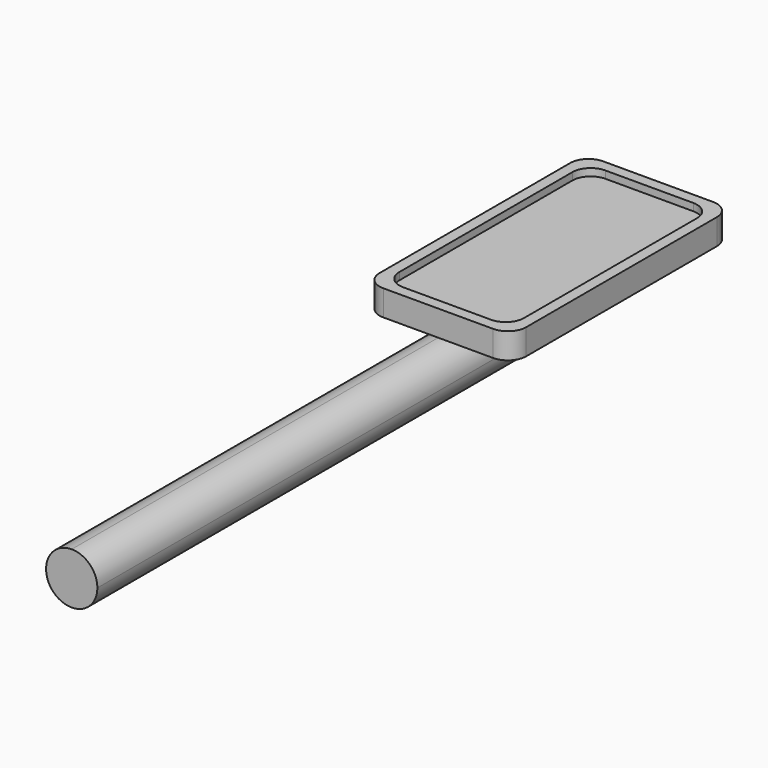
from build123d import *

# Parameters (mm, degrees)
F0_W     = 7
F0_H     = 200
F1_DEPTH = 7
F3_R     = 6.99999
F5_W     = 34
F5_H     = 69
F6_DEPTH = 5
F5_W_2   = 40
F5_H_2   = 75
F7_DEPTH = 7
F8_R     = 5
F9_R     = 5
F10_R    = 5
F11_R    = 5


# Not quite as in the source:
# - a fillet or chamfer is up to 0.001 mm smaller than in the source, because OpenCascade refuses the exact size


with BuildPart() as f1:
    # F0 (on Top) → F1 (new body)
    with BuildSketch(Plane.XY):
        with Locations((3.5, 0)):
            Rectangle(F0_W, F0_H)
    extrude(amount=F1_DEPTH)

    # F0 (on Top) → F2 (revolve)
    with BuildSketch(Plane.XY):
        with Locations((3.5, 0)):
            Rectangle(F0_W, F0_H)
    revolve(axis=Axis((0, 0, 0), (0, -1, 0)))

    # F3 (radius 7 in the source; OpenCascade refuses exactly that, so slightly less here)
    f3_edges = [f1.edges().sort_by_distance(p)[0] for p in [
        (7, 0, 7),
    ]]
    fillet(f3_edges, radius=F3_R)


with BuildPart() as f6:
    # F5 (on offset) → F6 (new body)
    with BuildSketch(Plane.XY.offset(7)):
        with Locations((0, 62.5)):
            Rectangle(F5_W, F5_H)
    extrude(amount=F6_DEPTH)


with BuildPart() as f7:
    # F5 (on offset) → F7 (new body)
    with BuildSketch(Plane.XY.offset(7)):
        with Locations((0, 62.5)):
            Rectangle(F5_W_2, F5_H_2)
        with Locations((0, 62.5)):
            Rectangle(F5_W, F5_H, mode=Mode.SUBTRACT)
    extrude(amount=F7_DEPTH)

    # F8
    f8_edges = [f7.edges().sort_by_distance(p)[0] for p in [
        (-17, 97, 10.5),
        (17, 28, 10.5),
        (-17, 28, 10.5),
    ]]
    fillet(f8_edges, radius=F8_R)

    # F9
    f9_edges = [f7.edges().sort_by_distance(p)[0] for p in [
        (17, 97, 10.5),
    ]]
    fillet(f9_edges, radius=F9_R)

    # F10
    f10_edges = [f7.edges().sort_by_distance(p)[0] for p in [
        (-20, 25, 10.5),
        (20, 25, 10.5),
    ]]
    fillet(f10_edges, radius=F10_R)

    # F11
    f11_edges = [f7.edges().sort_by_distance(p)[0] for p in [
        (20, 100, 10.5),
        (-20, 100, 10.5),
    ]]
    fillet(f11_edges, radius=F11_R)


solid = Compound([f1.part, f6.part, f7.part])
